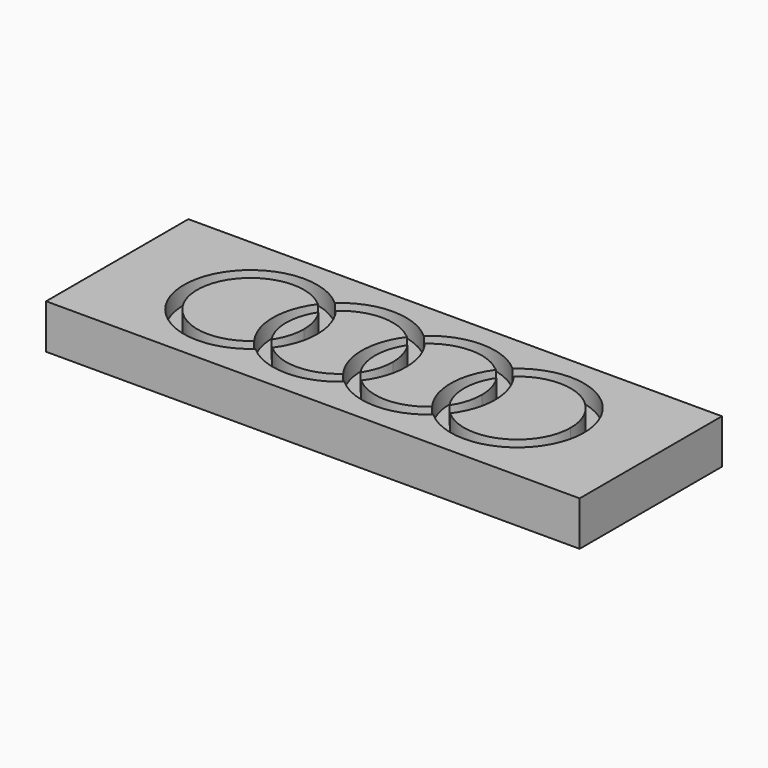
from build123d import *

# Parameters (mm, degrees)
F0_W     = 60
F0_H     = 20
F1_DEPTH = 5
F3_DEPTH = 2


with BuildPart() as f1:
    # F0 (on Top) → F1 (new body)
    with BuildSketch(Plane.XY):
        Rectangle(F0_W, F0_H)
    extrude(amount=F1_DEPTH)

    # F2 (on face) → F3 (cut)
    with BuildSketch(Plane.XY.offset(5)):
        with BuildLine():
            ThreePointArc((-8.9875, -4.4832849285), (-7.8815819875, -2.3618054535), (-7.5, 0))
            ThreePointArc((-7.5, 0), (-7.8815819875, 2.3618054535), (-8.9875, 4.4832849285))
            ThreePointArc((-8.9875, 4.4832849285), (-9.5314526404, 3.9326755483), (-10, 3.3166247904))
            ThreePointArc((-10, 3.3166247904), (-9.2554373535, 1.7320508076), (-9, 0))
            ThreePointArc((-9, 0), (-9.2554373535, -1.7320508076), (-10, -3.3166247904))
            ThreePointArc((-10, -3.3166247904), (-9.5314526404, -3.9326755483), (-8.9875, -4.4832849285))
        make_face()
        with BuildLine():
            ThreePointArc((-10, 3.3166247904), (-9.5314526404, 3.9326755483), (-8.9875, 4.4832849285))
            ThreePointArc((-8.9875, 4.4832849285), (-9.4660061735, 5.0621055232), (-10, 5.5901699437))
            ThreePointArc((-10, 5.5901699437), (-10.5339938265, 5.0621055232), (-11.0125, 4.4832849285))
            ThreePointArc((-11.0125, 4.4832849285), (-10.4685473596, 3.9326755483), (-10, 3.3166247904))
        make_face()
        with BuildLine():
            ThreePointArc((-10, 5.5901699437), (-9.4660061735, 5.0621055232), (-8.9875, 4.4832849285))
            ThreePointArc((-8.9875, 4.4832849285), (-5, 6), (-1.0125, 4.4832849285))
            ThreePointArc((-1.0125, 4.4832849285), (-0.5339938265, 5.0621055232), (0, 5.5901699437))
            ThreePointArc((0, 5.5901699437), (-5, 7.5), (-10, 5.5901699437))
        make_face()
        with BuildLine():
            ThreePointArc((-1.0125, -4.4832849285), (-5, -6), (-8.9875, -4.4832849285))
            ThreePointArc((-8.9875, -4.4832849285), (-9.4660061735, -5.0621055232), (-10, -5.5901699437))
            ThreePointArc((-10, -5.5901699437), (-5, -7.5), (0, -5.5901699437))
            ThreePointArc((0, -5.5901699437), (-0.5339938265, -5.0621055232), (-1.0125, -4.4832849285))
        make_face()
        with BuildLine():
            ThreePointArc((-10, -5.5901699437), (-9.4660061735, -5.0621055232), (-8.9875, -4.4832849285))
            ThreePointArc((-8.9875, -4.4832849285), (-9.5314526404, -3.9326755483), (-10, -3.3166247904))
            ThreePointArc((-10, -3.3166247904), (-10.4685473596, -3.9326755483), (-11.0125, -4.4832849285))
            ThreePointArc((-11.0125, -4.4832849285), (-10.5339938265, -5.0621055232), (-10, -5.5901699437))
        make_face()
        with BuildLine():
            ThreePointArc((-11.0125, 4.4832849285), (-10.5339938265, 5.0621055232), (-10, 5.5901699437))
            ThreePointArc((-10, 5.5901699437), (-22.5, 0), (-10, -5.5901699437))
            ThreePointArc((-10, -5.5901699437), (-10.5339938265, -5.0621055232), (-11.0125, -4.4832849285))
            ThreePointArc((-11.0125, -4.4832849285), (-21, 0), (-11.0125, 4.4832849285))
        make_face()
        with BuildLine():
            ThreePointArc((0, 5.5901699437), (-0.5339938265, 5.0621055232), (-1.0125, 4.4832849285))
            ThreePointArc((-1.0125, 4.4832849285), (-0.4685473596, 3.9326755483), (0, 3.3166247904))
            ThreePointArc((0, 3.3166247904), (0.4685473596, 3.9326755483), (1.0125, 4.4832849285))
            ThreePointArc((1.0125, 4.4832849285), (0.5339938265, 5.0621055232), (0, 5.5901699437))
        make_face()
        with BuildLine():
            ThreePointArc((0, 3.3166247904), (-0.4685473596, 3.9326755483), (-1.0125, 4.4832849285))
            ThreePointArc((-1.0125, 4.4832849285), (-2.5, 0), (-1.0125, -4.4832849285))
            ThreePointArc((-1.0125, -4.4832849285), (-0.4685473596, -3.9326755483), (0, -3.3166247904))
            ThreePointArc((0, -3.3166247904), (-1, 0), (0, 3.3166247904))
        make_face()
        with BuildLine():
            ThreePointArc((-10, -3.3166247904), (-11, 0), (-10, 3.3166247904))
            ThreePointArc((-10, 3.3166247904), (-10.4685473596, 3.9326755483), (-11.0125, 4.4832849285))
            ThreePointArc((-11.0125, 4.4832849285), (-12.5, 0), (-11.0125, -4.4832849285))
            ThreePointArc((-11.0125, -4.4832849285), (-10.4685473596, -3.9326755483), (-10, -3.3166247904))
        make_face()
        with BuildLine():
            ThreePointArc((0, -3.3166247904), (-0.4685473596, -3.9326755483), (-1.0125, -4.4832849285))
            ThreePointArc((-1.0125, -4.4832849285), (-0.5339938265, -5.0621055232), (0, -5.5901699437))
            ThreePointArc((0, -5.5901699437), (0.5339938265, -5.0621055232), (1.0125, -4.4832849285))
            ThreePointArc((1.0125, -4.4832849285), (0.4685473596, -3.9326755483), (0, -3.3166247904))
        make_face()
        with BuildLine():
            ThreePointArc((10, 5.5901699437), (5, 7.5), (0, 5.5901699437))
            ThreePointArc((0, 5.5901699437), (0.5339938265, 5.0621055232), (1.0125, 4.4832849285))
            ThreePointArc((1.0125, 4.4832849285), (5, 6), (8.9875, 4.4832849285))
            ThreePointArc((8.9875, 4.4832849285), (9.4660061735, 5.0621055232), (10, 5.5901699437))
        make_face()
        with BuildLine():
            ThreePointArc((1.0125, 4.4832849285), (0.4685473596, 3.9326755483), (0, 3.3166247904))
            ThreePointArc((0, 3.3166247904), (0.7445626465, 1.7320508076), (1, 0))
            ThreePointArc((1, 0), (0.7445626465, -1.7320508076), (0, -3.3166247904))
            ThreePointArc((0, -3.3166247904), (0.4685473596, -3.9326755483), (1.0125, -4.4832849285))
            ThreePointArc((1.0125, -4.4832849285), (2.1184180125, -2.3618054535), (2.5, 0))
            ThreePointArc((2.5, 0), (2.1184180125, 2.3618054535), (1.0125, 4.4832849285))
        make_face()
        with BuildLine():
            ThreePointArc((1.0125, -4.4832849285), (0.5339938265, -5.0621055232), (0, -5.5901699437))
            ThreePointArc((0, -5.5901699437), (5, -7.5), (10, -5.5901699437))
            ThreePointArc((10, -5.5901699437), (9.4660061735, -5.0621055232), (8.9875, -4.4832849285))
            ThreePointArc((8.9875, -4.4832849285), (5, -6), (1.0125, -4.4832849285))
        make_face()
        with BuildLine():
            ThreePointArc((22.5, 0), (18.0618621785, 6.8465319688), (10, 5.5901699437))
            ThreePointArc((10, 5.5901699437), (10.5339938265, 5.0621055232), (11.0125, 4.4832849285))
            ThreePointArc((11.0125, 4.4832849285), (17.4571324751, 5.4738012386), (21, 0))
            ThreePointArc((21, 0), (17.4571324751, -5.4738012386), (11.0125, -4.4832849285))
            ThreePointArc((11.0125, -4.4832849285), (10.5339938265, -5.0621055232), (10, -5.5901699437))
            ThreePointArc((10, -5.5901699437), (18.0618621785, -6.8465319688), (22.5, 0))
        make_face()
        with BuildLine():
            ThreePointArc((11.0125, 4.4832849285), (10.5339938265, 5.0621055232), (10, 5.5901699437))
            ThreePointArc((10, 5.5901699437), (9.4660061735, 5.0621055232), (8.9875, 4.4832849285))
            ThreePointArc((8.9875, 4.4832849285), (9.5314526404, 3.9326755483), (10, 3.3166247904))
            ThreePointArc((10, 3.3166247904), (10.4685473596, 3.9326755483), (11.0125, 4.4832849285))
        make_face()
        with BuildLine():
            ThreePointArc((8.9875, -4.4832849285), (9.4660061735, -5.0621055232), (10, -5.5901699437))
            ThreePointArc((10, -5.5901699437), (10.5339938265, -5.0621055232), (11.0125, -4.4832849285))
            ThreePointArc((11.0125, -4.4832849285), (10.4685473596, -3.9326755483), (10, -3.3166247904))
            ThreePointArc((10, -3.3166247904), (9.5314526404, -3.9326755483), (8.9875, -4.4832849285))
        make_face()
        with BuildLine():
            ThreePointArc((10, 3.3166247904), (9.5314526404, 3.9326755483), (8.9875, 4.4832849285))
            ThreePointArc((8.9875, 4.4832849285), (7.5, 0), (8.9875, -4.4832849285))
            ThreePointArc((8.9875, -4.4832849285), (9.5314526404, -3.9326755483), (10, -3.3166247904))
            ThreePointArc((10, -3.3166247904), (9, 0), (10, 3.3166247904))
        make_face()
        with BuildLine():
            ThreePointArc((12.5, 0), (12.1184180125, 2.3618054535), (11.0125, 4.4832849285))
            ThreePointArc((11.0125, 4.4832849285), (10.4685473596, 3.9326755483), (10, 3.3166247904))
            ThreePointArc((10, 3.3166247904), (10.7445626465, 1.7320508076), (11, 0))
            ThreePointArc((11, 0), (10.7445626465, -1.7320508076), (10, -3.3166247904))
            ThreePointArc((10, -3.3166247904), (10.4685473596, -3.9326755483), (11.0125, -4.4832849285))
            ThreePointArc((11.0125, -4.4832849285), (12.1184180125, -2.3618054535), (12.5, 0))
        make_face()
    extrude(amount=-F3_DEPTH, mode=Mode.SUBTRACT)


solid = f1.part
